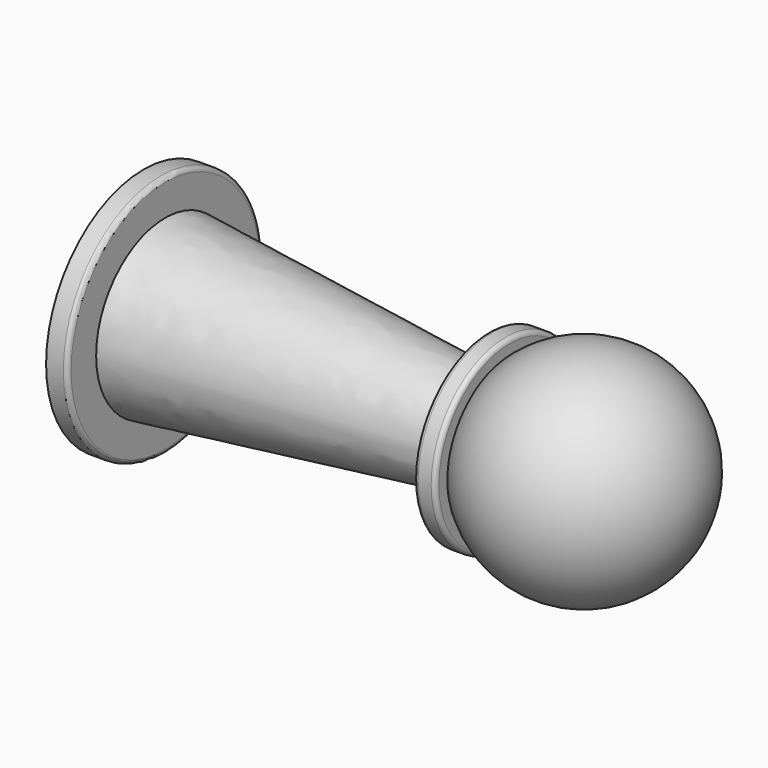
from build123d import *

# Parameters (mm, degrees)
F2_R      = 109.3978
F2_R_2    = 58.6042270255
F5_DEPTH  = 25.4
F4_R      = 101.6
F1_FACE_R = 58.6042270255
F7_R      = 5.08
F8_R      = 143.5389342848
F8_R_2    = 101.6000641099
F9_DEPTH  = 25.4
F10_R     = 5.08


with BuildPart() as f1:
    # F0 (on Front) → F1 (revolve)
    with BuildSketch(Plane.XZ):
        with BuildLine():
            ThreePointArc((-286.7686450481, 209.979994576), (-143.9331883211, 145.2187101443), (-47.0985754877, 268.5842216015))
            Line((-47.0985754877, 268.5842216015), (-286.7686450481, 268.5842216015))
            Line((-286.7686450481, 268.5842216015), (-286.7686450481, 209.979994576))
        make_face()
    revolve(axis=Axis((-174.0985754877, 0, 268.5842216015), (-1, 0, 0)))


with BuildPart() as f5:
    # F2 (on face) → F5 (new body)
    with BuildSketch(Plane(origin=(-286.7686450481, 0, 0), x_dir=(0, -1, 0), z_dir=(-1, 0, 0))):
        with Locations((0, 268.5842216015)):
            Circle(F2_R)
        with Locations((0, 268.5842216015)):
            Circle(F2_R_2, mode=Mode.SUBTRACT)
    extrude(amount=-F5_DEPTH)

    # F7
    f7_edges = [f5.edges().sort_by_distance(p)[0] for p in [
        (-261.368645, 109.3978, 268.584222),
        (-286.768645, 109.3978, 268.584222),
    ]]
    fillet(f7_edges, radius=F7_R)


with BuildPart() as f6:
    # F4 (on offset) → F6 section 0
    with BuildSketch(Plane(origin=(-667.7686450481, 0, 0), x_dir=(0, -1, 0), z_dir=(-1, 0, 0))):
        with Locations((-0.9220663342, 269.1939473152)):
            Circle(F4_R)
    # F1_face (on face) → F6 section 1
    with BuildSketch(Plane(origin=(-286.7686450481, 0, 268.5842216015), x_dir=(0, -1, 0), z_dir=(-1, 0, 0))):
        Circle(F1_FACE_R)
    loft()


with BuildPart() as f9:
    # F8 (on face) → F9 (new body)
    with BuildSketch(Plane(origin=(-667.7686450481, 0, 0), x_dir=(0, -1, 0), z_dir=(-1, 0, 0))):
        with Locations((-0.9220611856, 269.1939344642)):
            Circle(F8_R)
        with Locations((-0.9220611856, 269.1939344642)):
            Circle(F8_R_2, mode=Mode.SUBTRACT)
        with Locations((-0.9220611856, 269.1939344642)):
            Circle(F8_R_2)
    extrude(amount=F9_DEPTH)

    # F10
    f10_edges = [f9.edges().sort_by_distance(p)[0] for p in [
        (-667.768645, 144.460995, 269.193934),
    ]]
    fillet(f10_edges, radius=F10_R)


solid = Compound([f1.part, f5.part, f6.part, f9.part])
